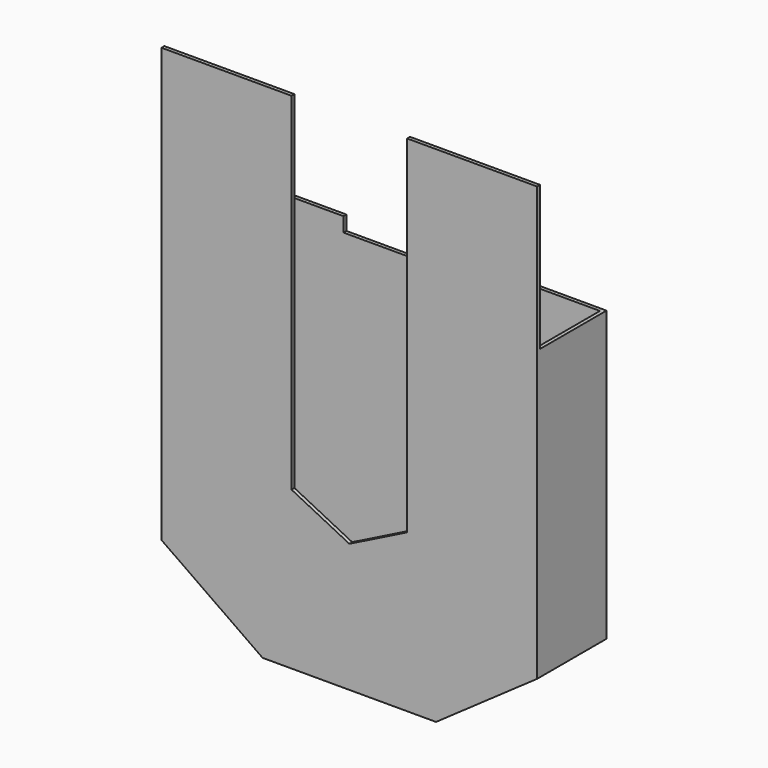
from build123d import *

# Parameters (mm, degrees)
F1_DEPTH  = 76.2
F2_T      = -3.175
F4_DEPTH  = 25.4
F5_W      = 127
F5_H      = 25.4
F6_DEPTH  = 25.4
F7_W      = 330.2
F7_H      = 127
F8_DEPTH  = 3.175
F9_W      = 101.6
F9_H      = 127
F10_DEPTH = 25.4


# Not quite as in the source:
# - a pattern or mirror of a feature is missing from the dataset's text; its kind, count and spacing are read off the source's solid


with BuildPart() as f1:
    # F0 (on Front) → F1 (new body)
    with BuildSketch(Plane.XZ):
        with BuildLine():
            ThreePointArc((-1.539e-07, -127), (89.8025611563, -89.8025612651), (127, 0))
            ThreePointArc((127, 0), (89.8025612186, 89.8025612028), (2.24e-08, 127))
            ThreePointArc((2.24e-08, 127), (-127, 8.82e-08), (-1.539e-07, -127))
        make_face()
        with BuildLine():
            ThreePointArc((2.24e-08, 127), (89.8025612186, 89.8025612028), (127, 0))
            ThreePointArc((127, 0), (89.8025611563, -89.8025612651), (-1.539e-07, -127))
            Line((-1.539e-07, -127), (165.1, -127))
            Line((165.1, -127), (165.1, 127))
            Line((165.1, 127), (2.24e-08, 127))
        make_face()
        with BuildLine():
            ThreePointArc((-1.539e-07, -127), (-127, 8.82e-08), (2.24e-08, 127))
            Line((2.24e-08, 127), (-165.1, 127))
            Line((-165.1, 127), (-165.1, -127))
            Line((-165.1, -127), (-1.539e-07, -127))
        make_face()
        Polygon((165.1, -127), (-1.539e-07, -127), (-165.1, -127), (-76.2, -189.2484501468), (76.2, -189.2484501468), align=None)
    extrude(amount=F1_DEPTH)

    # F2
    f2_openings = [f1.faces().sort_by_distance(p)[0] for p in [
        (0, -38.1, 127),
    ]]
    offset(amount=F2_T, openings=f2_openings)

    # F3 (on face) → F4 (cut)
    with BuildSketch(Plane.XZ.offset(76.2)):
        Polygon((0, -76.2), (0, 127), (-50.8, 127), (-50.8, -50.8), align=None)
    f4 = extrude(amount=-F4_DEPTH, mode=Mode.SUBTRACT)

    # F4_copies: F4 across plane
    add(f4.mirror(Plane(origin=(0, 0, 0), x_dir=(0, 0, 1), z_dir=(1, 0, 0))), mode=Mode.SUBTRACT)

    # F5 (on face) → F6 (cut)
    with BuildSketch(Plane.XZ.offset(3.175)):
        with Locations((0, 127)):
            Rectangle(F5_W, F5_H)
    extrude(amount=-F6_DEPTH, mode=Mode.SUBTRACT)

    # F7 (on face) → F8 (join)
    with BuildSketch(Plane.XZ.offset(76.2)):
        with Locations((0, 190.5)):
            Rectangle(F7_W, F7_H)
    extrude(amount=-F8_DEPTH)

    # F9 (on face) → F10 (cut)
    with BuildSketch(Plane.XZ.offset(76.2)):
        with Locations((0, 190.5)):
            Rectangle(F9_W, F9_H)
    extrude(amount=-F10_DEPTH, mode=Mode.SUBTRACT)


solid = f1.part
